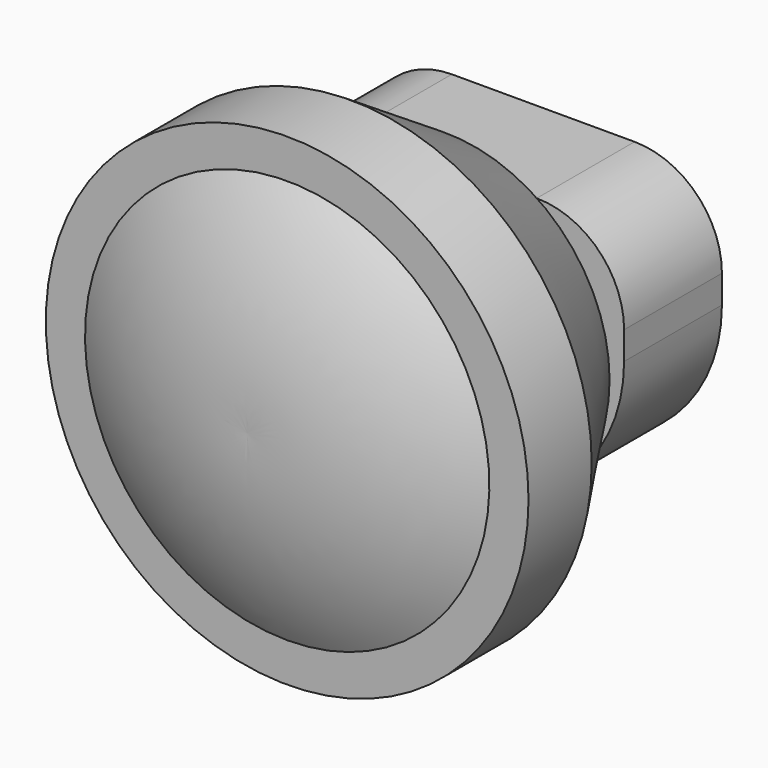
from build123d import *

# Parameters (mm, degrees)
F0_R     = 1.2446
F0_R_2   = 8.636
F1_DEPTH = 8.89
F0_R_3   = 8.509
F2_DEPTH = 3.175
F3_R     = 11.938
F4_DEPTH = 8.636
F4_TAPER = -33
F5_R     = 17.54632
F5_R_2   = 14.5791622743
F6_DEPTH = 5.7404


with BuildPart() as f1:
    # F0 (on Front) → F1 (new body)
    with BuildSketch(Plane.XZ):
        with BuildLine():
            Line((6.6421, 9.906), (-6.6421, 9.906))
            ThreePointArc((-6.6421, 9.906), (-11.1322280605, 8.0461280605), (-12.9921, 3.556))
            Line((-12.9921, 3.556), (-12.9921, 1.524))
            ThreePointArc((-12.9921, 1.524), (-9.644330509, -6.558230509), (-1.5621, -9.906))
            Line((-1.5621, -9.906), (1.5621, -9.906))
            ThreePointArc((1.5621, -9.906), (9.644330509, -6.558230509), (12.9921, 1.524))
            Line((12.9921, 1.524), (12.9921, 3.556))
            ThreePointArc((12.9921, 3.556), (11.1322280605, 8.0461280605), (6.6421, 9.906))
        make_face()
        with Locations((-10.4775, 0)):
            Circle(F0_R, mode=Mode.SUBTRACT)
        Circle(F0_R_2, mode=Mode.SUBTRACT)
        with Locations((10.4775, 0)):
            Circle(F0_R, mode=Mode.SUBTRACT)
    extrude(amount=F1_DEPTH)

    # F0 (on Front) → F2 (join)
    with BuildSketch(Plane.XZ):
        Circle(F0_R_2)
        Circle(F0_R_3, mode=Mode.SUBTRACT)
    extrude(amount=F2_DEPTH)


with BuildPart() as f4:
    # F3 (on face) → F4 (new body)
    with BuildSketch(Plane.XZ.offset(8.89)):
        Circle(F3_R)
    extrude(amount=F4_DEPTH, taper=F4_TAPER)

    # F5 (on face) → F6 (join)
    with BuildSketch(Plane.XZ.offset(17.526)):
        Circle(F5_R)
        Circle(F5_R_2, mode=Mode.SUBTRACT)
    extrude(amount=F6_DEPTH)

    # F7 (on Right) → F8 (revolve)
    with BuildSketch(Plane.YZ):
        with BuildLine():
            Line((-23.2664, 0), (-26.8908049911, 0))
            ThreePointArc((-26.8908049911, 0), (-26.1383181436, -7.6104076675), (-23.2664, -14.6981878206))
            Line((-23.2664, -14.6981878206), (-23.2664, 0))
        make_face()
    revolve(axis=Axis((0, -25.0786024956, 0), (0, -1, 0)))


solid = Compound([f1.part, f4.part])
